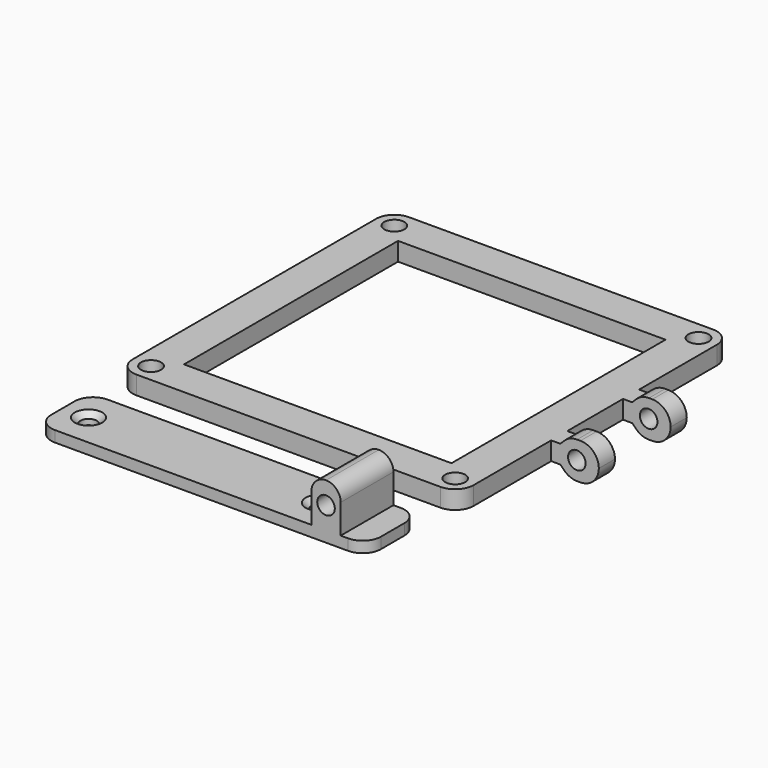
from build123d import *

# Parameters (mm, degrees)
F0_W          = 90
F0_H          = 18
F0_R          = 2.25
F1_DEPTH      = 3
F2_W          = 8
F2_H          = 18
F3_DEPTH      = 12
F4_R          = 2.4
F5_DEPTH      = 18
F6_SIZE       = 1.5
F7_W          = 93
F7_H          = 93
F7_R          = 2.75
F7_W_2        = 73
F7_H_2        = 73
F8_DEPTH      = 5
F9_W          = 5.5
F9_H          = 5
F9_H_2        = 2.5
F10_DEPTH     = 13
F11_R         = 2.4
F12_DEPTH     = 89.3579660494
F13_T4_DEPTH  = 31.2168298797
F13_T9_DEPTH  = 31.2168298797
F13_T14_DEPTH = 31.2168298797
F13_T19_DEPTH = 31.2168298797
F14_R         = 4.99999
F15_R         = 5
F16_R         = 3.99999
F17_R         = 5


# Not quite as in the source:
# - a fillet or chamfer that OpenCascade refuses, or shapes differently, is made with other operations: its cross-section is extruded or revolved along the edge and cut away or added
# - a fillet or chamfer is up to 0.001 mm smaller than in the source, because OpenCascade refuses the exact size


with BuildPart() as f1:
    # F0 (on Top) → F1 (new body)
    with BuildSketch(Plane.XY):
        with Locations((3.3186358213, 0)):
            Rectangle(F0_W, F0_H)
        with Locations((-34.6813641787, 0)):
            Circle(F0_R, mode=Mode.SUBTRACT)
        with Locations((28.3186358213, 0)):
            Circle(F0_R, mode=Mode.SUBTRACT)
    extrude(amount=F1_DEPTH)

    # F2 (on face) → F3 (join)
    with BuildSketch(Plane.XY.offset(3)):
        with Locations((37.3186358213, 0)):
            Rectangle(F2_W, F2_H)
    extrude(amount=F3_DEPTH)

    # F4 (on face) → F5 (cut, through all)
    with BuildSketch(Plane(origin=(0, 9, 0), x_dir=(-1, 0, 0), z_dir=(0, 1, 0))):
        with Locations((-37.3186358213, 9)):
            Circle(F4_R)
    extrude(amount=-F5_DEPTH, mode=Mode.SUBTRACT)

    # F6
    f6_edges = [f1.edges().sort_by_distance(p)[0] for p in [
        (-36.931364, 0, 3),
        (26.068636, 0, 3),
    ]]
    chamfer(f6_edges, length=F6_SIZE)

    # F16 (radius 4 in the source; OpenCascade refuses exactly that, so slightly less here)
    f16_edges = [f1.edges().sort_by_distance(p)[0] for p in [
        (41.318636, 0, 15),
        (33.318636, 0, 15),
    ]]
    fillet(f16_edges, radius=F16_R)

    # F17
    f17_edges = [f1.edges().sort_by_distance(p)[0] for p in [
        (-41.681364, -9, 1.5),
        (-41.681364, 9, 1.5),
        (48.318636, -9, 1.5),
        (48.318636, 9, 1.5),
    ]]
    fillet(f17_edges, radius=F17_R)


with BuildPart() as f8:
    # F7 (on Top) → F8 (new body)
    with BuildSketch(Plane.XY):
        with Locations((4.7773654461, 65.3569660494)):
            Rectangle(F7_W, F7_H)
        with Locations((-36.7226345539, 23.8569660494)):
            Circle(F7_R, mode=Mode.SUBTRACT)
        with Locations((46.2773654461, 23.8569660494)):
            Circle(F7_R, mode=Mode.SUBTRACT)
        with Locations((4.7773654461, 65.3569660494)):
            Rectangle(F7_W_2, F7_H_2, mode=Mode.SUBTRACT)
        with Locations((-36.7226345539, 106.8569660494)):
            Circle(F7_R, mode=Mode.SUBTRACT)
        with Locations((46.2773654461, 106.8569660494)):
            Circle(F7_R, mode=Mode.SUBTRACT)
    extrude(amount=F8_DEPTH)

    # F9 (on face) → F10 (join)
    with BuildSketch(Plane.YZ.offset(51.2773654461)):
        with Locations((53.1069660494, 2.5)):
            Rectangle(F9_W, F9_H)
        with Locations((53.1069660494, -1.25)):
            Rectangle(F9_W, F9_H_2)
        with Locations((77.6069660494, 6.25)):
            Rectangle(F9_W, F9_H_2)
        with Locations((77.6069660494, -1.25)):
            Rectangle(F9_W, F9_H_2)
        with Locations((77.6069660494, 2.5)):
            Rectangle(F9_W, F9_H)
        with Locations((53.1069660494, 6.25)):
            Rectangle(F9_W, F9_H_2)
    extrude(amount=F10_DEPTH)

    # F11 (on face) → F12 (cut, through all)
    with BuildSketch(Plane(origin=(0, 80.3569660494, 0), x_dir=(-1, 0, 0), z_dir=(0, 1, 0))):
        with Locations((-58.2773654461, 2.5)):
            Circle(F11_R)
    extrude(amount=-F12_DEPTH, mode=Mode.SUBTRACT)

    # F13: chamfer of 5 on 4 edges, made by hand


with BuildPart() as f13_tool2:
    # F13_s3 → F13_t4 (new body)
    with BuildSketch(Plane.XZ.offset(-68.7153809892)):
        Polygon((51.2773654461, 2.5), (56.2773654461, 7.5), (51.2773654461, 7.5), align=None)
    extrude(amount=F13_T4_DEPTH)

    split(bisect_by=Plane.XY.offset(5), keep=Keep.TOP)


with BuildPart() as f8_1:
    add(f8.part)

    # F13_t1: cut F13_tool2
    add(f13_tool2.part, mode=Mode.SUBTRACT)


with BuildPart() as f13_tool7:
    # F13_s8 → F13_t9 (new body)
    with BuildSketch(Plane.XZ.offset(-93.2153809892)):
        Polygon((51.2773654461, 2.5), (56.2773654461, 7.5), (51.2773654461, 7.5), align=None)
    extrude(amount=F13_T9_DEPTH)

    split(bisect_by=Plane.XY.offset(5), keep=Keep.TOP)


with BuildPart() as f8_2:
    add(f8_1.part)

    # F13_t6: cut F13_tool7
    add(f13_tool7.part, mode=Mode.SUBTRACT)


with BuildPart() as f13_tool12:
    # F13_s13 → F13_t14 (new body)
    with BuildSketch(Plane.XZ.offset(-37.4985511096)):
        Polygon((51.2773654461, 2.5), (56.2773654461, -2.5), (51.2773654461, -2.5), align=None)
    extrude(amount=-F13_T14_DEPTH)

    split(bisect_by=Plane.XY, keep=Keep.BOTTOM)


with BuildPart() as f8_3:
    add(f8_2.part)

    # F13_t11: cut F13_tool12
    add(f13_tool12.part, mode=Mode.SUBTRACT)


with BuildPart() as f13_tool17:
    # F13_s18 → F13_t19 (new body)
    with BuildSketch(Plane.XZ.offset(-61.9985511096)):
        Polygon((51.2773654461, 2.5), (56.2773654461, -2.5), (51.2773654461, -2.5), align=None)
    extrude(amount=-F13_T19_DEPTH)

    split(bisect_by=Plane.XY, keep=Keep.BOTTOM)


with BuildPart() as f8_4:
    add(f8_3.part)

    # F13_t16: cut F13_tool17
    add(f13_tool17.part, mode=Mode.SUBTRACT)

    # F14 (radius 5 in the source; OpenCascade refuses exactly that, so slightly less here)
    f14_edges = [f8_4.edges().sort_by_distance(p)[0] for p in [
        (64.277365, 53.106966, 7.5),
        (64.277365, 77.606966, 7.5),
        (64.277365, 77.606966, -2.5),
        (64.277365, 53.106966, -2.5),
        (56.277365, 53.106966, 7.5),
        (56.277365, 53.106966, -2.5),
        (56.277365, 77.606966, -2.5),
        (56.277365, 77.606966, 7.5),
    ]]
    fillet(f14_edges, radius=F14_R)

    # F15
    f15_edges = [f8_4.edges().sort_by_distance(p)[0] for p in [
        (51.277365, 18.856966, 2.5),
        (51.277365, 111.856966, 2.5),
        (-41.722635, 111.856966, 2.5),
        (-41.722635, 18.856966, 2.5),
    ]]
    fillet(f15_edges, radius=F15_R)


solid = Compound([f1.part, f8_4.part])
